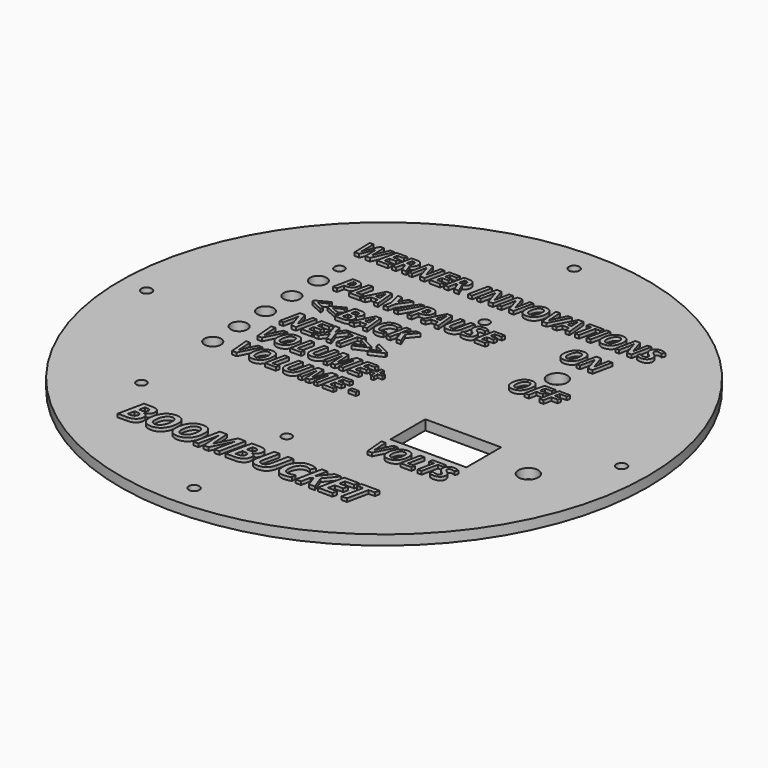
from build123d import *

# Parameters (mm, degrees)
F0_R           = 80
F0_R_2         = 1.5
F0_R_3         = 2.5
F1_DEPTH       = 3
F2_R           = 3
F2_W           = 23
F2_H           = 13.1896547973
F4_DEPTH       = 3
F3_TEXT_SIZE   = 8.3333333333
F3_TEXT_SIZE_2 = 8.3512937029
F3_TEXT_SIZE_3 = 8.6206891057
F5_DEPTH       = 1
F6_TEXT_SIZE   = 8.3333333333
F7_DEPTH       = 1
F8_TEXT_SIZE   = 11.0420784766
F8_TEXT_SIZE_2 = 8.3333333333
F9_DEPTH       = 1
F10_R          = 1.6
F11_DEPTH      = 3


# Not quite as in the source:
# - Text() gives the source's letters only with a copy of the font that has no kerning and outlines rounded to 1/6400 em; it was checked with that copy


with BuildPart() as f1:
    # F0 (on Top) → F1 (new body)
    with BuildSketch(Plane.XY):
        Circle(F0_R)
        with Locations((-43.4069000185, -37.6550041139)):
            Circle(F0_R_2, mode=Mode.SUBTRACT)
        with Locations((-43.4069000185, -10.6550041139)):
            Circle(F0_R_3, mode=Mode.SUBTRACT)
        with Locations((-43.4069000185, -0.6550041139)):
            Circle(F0_R_3, mode=Mode.SUBTRACT)
        with Locations((0.5930999815, -37.6550041139)):
            Circle(F0_R_2, mode=Mode.SUBTRACT)
        with Locations((-43.4069000185, 9.3449958861)):
            Circle(F0_R_3, mode=Mode.SUBTRACT)
        with Locations((-43.4069000185, 19.3449958861)):
            Circle(F0_R_3, mode=Mode.SUBTRACT)
        with Locations((-43.4069000185, 29.3449958861)):
            Circle(F0_R_3, mode=Mode.SUBTRACT)
        with Locations((-43.4069000185, 37.3449958861)):
            Circle(F0_R_2, mode=Mode.SUBTRACT)
        with Locations((0.5930999815, 37.3449958861)):
            Circle(F0_R_2, mode=Mode.SUBTRACT)
    extrude(amount=F1_DEPTH)

    # F2 (on face) → F4 (cut)
    with BuildSketch(Plane.XY.offset(3)):
        with Locations((32.2074657083, 25.3846999258)):
            Circle(F2_R)
        with Locations((32.2074657083, -16.8750006706)):
            Rectangle(F2_W, F2_H)
        with Locations((57.2198294103, -16.8750006706)):
            Circle(F2_R)
    extrude(amount=-F4_DEPTH, mode=Mode.SUBTRACT)

    # F3 (on face) → F5 (join)
    with BuildSketch(Plane.XY.offset(3)):
        with Locations((-37.7999938541, 27.5999915494)):
            Text('PLAY/PAUSE', F3_TEXT_SIZE, font='Open Sans', font_style=FontStyle.BOLDITALIC, text_align=(TextAlign.LEFT, TextAlign.BOTTOM))
        with Locations((-37.1633744083, 16.0991381854)):
            Text('<<BACK', F3_TEXT_SIZE_2, font='Open Sans', font_style=FontStyle.BOLDITALIC, text_align=(TextAlign.LEFT, TextAlign.BOTTOM))
        with Locations((-36.7529614018, 6.0129314661)):
            Text('NEXT>>', F3_TEXT_SIZE_3, font='Open Sans', font_style=FontStyle.BOLDITALIC, text_align=(TextAlign.LEFT, TextAlign.BOTTOM))
        with Locations((-37.0474159718, -3.2844826989)):
            Text('VOLUME+', F3_TEXT_SIZE, font='Open Sans', font_style=FontStyle.BOLDITALIC, text_align=(TextAlign.LEFT, TextAlign.BOTTOM))
        with Locations((-36.9632720881, -12.9827586412)):
            Text('VOLUME -', F3_TEXT_SIZE, font='Open Sans', font_style=FontStyle.BOLDITALIC, text_align=(TextAlign.LEFT, TextAlign.BOTTOM))
    extrude(amount=F5_DEPTH)

    # F6 (on face) → F7 (join)
    with BuildSketch(Plane.XY.offset(3)):
        with Locations((25.9128484879, 32.611022843)):
            Text('ON', F6_TEXT_SIZE, font='Open Sans', font_style=FontStyle.BOLDITALIC, text_align=(TextAlign.LEFT, TextAlign.BOTTOM))
        with Locations((25.6841817166, 13.3094648421)):
            Text('OFF', F6_TEXT_SIZE, font='Open Sans', font_style=FontStyle.BOLDITALIC, text_align=(TextAlign.LEFT, TextAlign.BOTTOM))
        with Locations((20.1502805476, -33.0123332739)):
            Text('VOLTS', F6_TEXT_SIZE, font='Open Sans', font_style=FontStyle.BOLDITALIC, text_align=(TextAlign.LEFT, TextAlign.BOTTOM))
    extrude(amount=F7_DEPTH)

    # F8 (on face) → F9 (join)
    with BuildSketch(Plane.XY.offset(3)):
        with Locations((-37.0168427682, -55.0028945647)):
            Text('BOOMBUCKET', F8_TEXT_SIZE, font='Open Sans', font_style=FontStyle.BOLDITALIC, text_align=(TextAlign.LEFT, TextAlign.BOTTOM))
        with Locations((-45.55859375, 44.6319218487)):
            Text('WERNER INNOVATIONS', F8_TEXT_SIZE_2, font='Open Sans', font_style=FontStyle.BOLDITALIC, text_align=(TextAlign.LEFT, TextAlign.BOTTOM))
    extrude(amount=F9_DEPTH)

    # F10 (on face) → F11 (cut)
    with BuildSketch(Plane.XY.offset(3)):
        with Locations((0, 72)):
            Circle(F10_R)
        with Locations((0, -72)):
            Circle(F10_R)
        with Locations((72, 0)):
            Circle(F10_R)
        with Locations((-72, 0)):
            Circle(F10_R)
    extrude(amount=-F11_DEPTH, mode=Mode.SUBTRACT)


solid = f1.part
